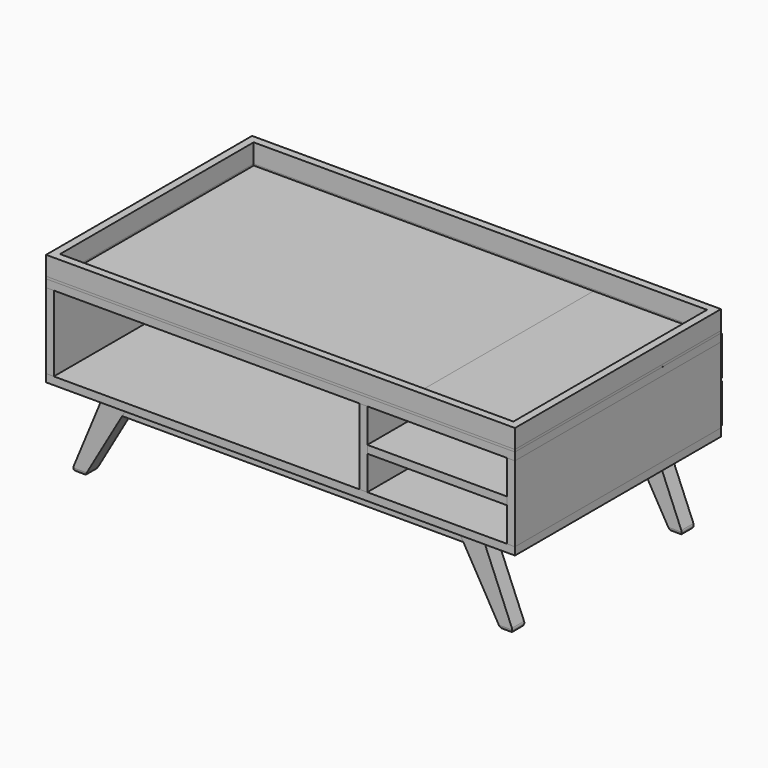
from build123d import *

# Parameters (mm, degrees)
F1_DEPTH       = 340.5
F1_DEPTH_BACK  = 340.5
F2_DEPTH       = 340.5
F2_DEPTH_BACK  = 340.5
F0_W           = 20.5
F0_H           = 200
F3_DEPTH       = 340.5
F3_DEPTH_BACK  = 340.5
F6_DEPTH       = 40
F7_R           = 10
F7_2_R         = 10
F8_DEPTH       = 40
F10_W          = 46.1880215352
F10_H          = 40
F11_DEPTH      = 520
F12_W          = 7
F12_H          = 96.75
F13_DEPTH      = 20
F14_W          = 1240
F14_H          = 681
F14_W_2        = 1230
F14_H_2        = 671
F14_W_3        = 1199
F14_H_3        = 640
F15_DEPTH      = 6
F16_W          = 898.5
F16_H          = 637
F17_DEPTH      = 3
F16_W_2        = 297.5
F18_DEPTH      = 3
F19_DEPTH      = 50
F22_DEPTH      = 370
F0_W_2         = 370
F0_H_2         = 20.5
F23_DEPTH      = 19.5
F23_DEPTH_BACK = 340.5


# Not quite as in the source:
# - a feature names something its author has since deleted; it is built from what else it names


with BuildPart() as f1:
    # F0 (on Front) → F1 (new body, two sides)
    with BuildSketch(Plane.XZ) as f1_sk:
        Polygon((-599.5, -220.5), (-620, -220.5), (-620, -241), (620, -241), (620, -220.5), (599.5, -220.5), (229.5, -220.5), (209, -220.5), align=None)
    extrude(amount=F1_DEPTH)
    extrude(f1_sk.sketch, amount=-F1_DEPTH_BACK)


with BuildPart() as f2:
    # F0 (on Front) → F2 (new body, two sides)
    with BuildSketch(Plane.XZ) as f2_sk:
        Polygon((229.5, -20.5), (209, -20.5), (209, -220.5), (229.5, -220.5), (229.5, -130.75), (229.5, -110.25), align=None)
    extrude(amount=F2_DEPTH)
    extrude(f2_sk.sketch, amount=-F2_DEPTH_BACK)


with BuildPart() as f2b:
    # F0 (on Front) → F2, piece 2 (new body, two sides)
    with BuildSketch(Plane.XZ) as f2_2_sk:
        with Locations((-609.75, -120.5)):
            Rectangle(F0_W, F0_H)
    extrude(amount=F2_DEPTH)
    extrude(f2_2_sk.sketch, amount=-F2_DEPTH_BACK)


with BuildPart() as f2c:
    # F0 (on Front) → F2, piece 3 (new body, two sides)
    with BuildSketch(Plane.XZ) as f2_3_sk:
        Polygon((620, -220.5), (620, -20.5), (599.5, -20.5), (599.5, -110.25), (599.5, -130.75), (599.5, -220.5), align=None)
    extrude(amount=F2_DEPTH)
    extrude(f2_3_sk.sketch, amount=-F2_DEPTH_BACK)


with BuildPart() as f3:
    # F0 (on Front) → F3 (new body, two sides)
    with BuildSketch(Plane.XZ) as f3_sk:
        Polygon((620, 0), (-620, 0), (-620, -20.5), (-599.5, -20.5), (209, -20.5), (229.5, -20.5), (599.5, -20.5), (620, -20.5), align=None)
    extrude(amount=F3_DEPTH)
    extrude(f3_sk.sketch, amount=-F3_DEPTH_BACK)


with BuildPart() as f6:
    # F5 (on offset) → F6 (new body)
    with BuildSketch(Plane.XZ.offset(260)):
        Polygon((-428.0310354944, -241), (-497.3130677972, -241), (-585.3589838486, -453.5), (-550.7179676972, -453.5), (-451.125046262, -281), align=None)
    extrude(amount=F6_DEPTH)

    # F7
    f7_edges = [f6.edges().sort_by_distance(p)[0] for p in [
        (-568.038476, -300, -453.5),
        (-550.717968, -280, -453.5),
        (-568.038476, -260, -453.5),
        (-585.358984, -280, -453.5),
    ]]
    fillet(f7_edges, radius=F7_R)


with BuildPart() as f6b:
    # F5 (on offset) → F6, piece 2 (new body)
    with BuildSketch(Plane.XZ.offset(260)):
        Polygon((497.3130677972, -241), (428.0310354944, -241), (451.125046262, -281), (550.7179676972, -453.5), (585.3589838486, -453.5), align=None)
    extrude(amount=F6_DEPTH)

    # F7#2
    f7_2_edges = [f6b.edges().sort_by_distance(p)[0] for p in [
        (568.038476, -300, -453.5),
        (550.717968, -280, -453.5),
        (568.038476, -260, -453.5),
        (585.358984, -280, -453.5),
    ]]
    fillet(f7_2_edges, radius=F7_2_R)


with BuildPart() as f8:
    # F5 (on offset) → F8 (new body)
    with BuildSketch(Plane.XZ.offset(260)):
        Polygon((428.0310354944, -241), (-428.0310354944, -241), (-451.125046262, -281), (451.125046262, -281), align=None)
    extrude(amount=F8_DEPTH)


with BuildPart() as f9_1:
    # F9: instance of F6
    add(f6.part.mirror(Plane.XZ))


with BuildPart() as f9_2:
    # F9: instance of F6b
    add(f6b.part.mirror(Plane.XZ))


with BuildPart() as f9_3:
    # F9: instance of F8
    add(f8.part.mirror(Plane.XZ))


with BuildPart() as f11:
    # F10 (on face) → F11 (new body, through all)
    with BuildSketch(Plane.XZ.offset(260)):
        with Locations((474.2190570296, -261)):
            Rectangle(F10_W, F10_H)
    extrude(amount=-F11_DEPTH)


with BuildPart() as f11b:
    # F10 (on face) → F11, piece 2 (new body, through all)
    with BuildSketch(Plane.XZ.offset(260)):
        with Locations((-474.2190570296, -261)):
            Rectangle(F10_W, F10_H)
    extrude(amount=-F11_DEPTH)


with BuildPart() as f13:
    # F12 (on face) → F13 (new body)
    with BuildSketch(Plane(origin=(0, 340.5, 0), x_dir=(-1, 0, 0), z_dir=(0, 1, 0))):
        with Locations((-603, -68.875)):
            Rectangle(F12_W, F12_H)
        Polygon((-222.5, -117.25), (-222.5, -13.5), (-606.5, -13.5), (-606.5, -20.5), (-599.5, -20.5), (-599.5, -117.25), align=None)
    extrude(amount=F13_DEPTH)


with BuildPart() as f13b:
    # F12 (on face) → F13, piece 2 (new body)
    with BuildSketch(Plane(origin=(0, 340.5, 0), x_dir=(-1, 0, 0), z_dir=(0, 1, 0))):
        with Locations((-603, -172.125)):
            Rectangle(F12_W, F12_H)
        Polygon((-222.5, -123.75), (-599.5, -123.75), (-599.5, -220.5), (-606.5, -220.5), (-606.5, -227.5), (-222.5, -227.5), align=None)
    extrude(amount=F13_DEPTH)


with BuildPart() as f15:
    # F14 (on face) → F15 (new body)
    with BuildSketch(Plane.XY):
        Rectangle(F14_W, F14_H)
        Rectangle(F14_W_2, F14_H_2, mode=Mode.SUBTRACT)
        Rectangle(F14_W_2, F14_H_2)
        Rectangle(F14_W_3, F14_H_3, mode=Mode.SUBTRACT)
    extrude(amount=F15_DEPTH)


with BuildPart() as f17:
    # F16 (on face) → F17 (new body)
    with BuildSketch(Plane.XY):
        with Locations((-148.75, 0)):
            Rectangle(F16_W, F16_H)
    extrude(amount=F17_DEPTH)


with BuildPart() as f18:
    # F16 (on face) → F18 (new body, through all)
    with BuildSketch(Plane.XY):
        with Locations((449.25, 0)):
            Rectangle(F16_W_2, F16_H)
    extrude(amount=F18_DEPTH)


with BuildPart() as f19:
    # F19 (new): a face of the model
    f19_faces = [f15.part.faces().sort_by_distance(p)[0] for p in [
        (-613.646946667, 0, 6),
    ]]
    extrude(f19_faces, amount=F19_DEPTH)


with BuildPart() as f22:
    # F21 (on face) → F22 (new body, through all)
    with BuildSketch(Plane.YZ.offset(229.5)):
        Polygon((40, -20.5), (19.5, -20.5), (19.5, -130.75), (19.5, -220.5), (40, -220.5), (40, -130.75), align=None)
    extrude(amount=F22_DEPTH)


with BuildPart() as f23:
    # F0 (on Front) → F23 (new body, two sides)
    with BuildSketch(Plane.XZ) as f23_sk:
        with Locations((414.5, -120.5)):
            Rectangle(F0_W_2, F0_H_2)
    extrude(amount=-F23_DEPTH)
    extrude(f23_sk.sketch, amount=F23_DEPTH_BACK)


solid = Compound([f1.part, f2.part, f2b.part, f2c.part, f3.part, f6.part, f6b.part, f8.part, f9_1.part, f9_2.part, f9_3.part, f11.part, f11b.part, f13.part, f13b.part, f15.part, f17.part, f18.part, f19.part, f22.part, f23.part])
